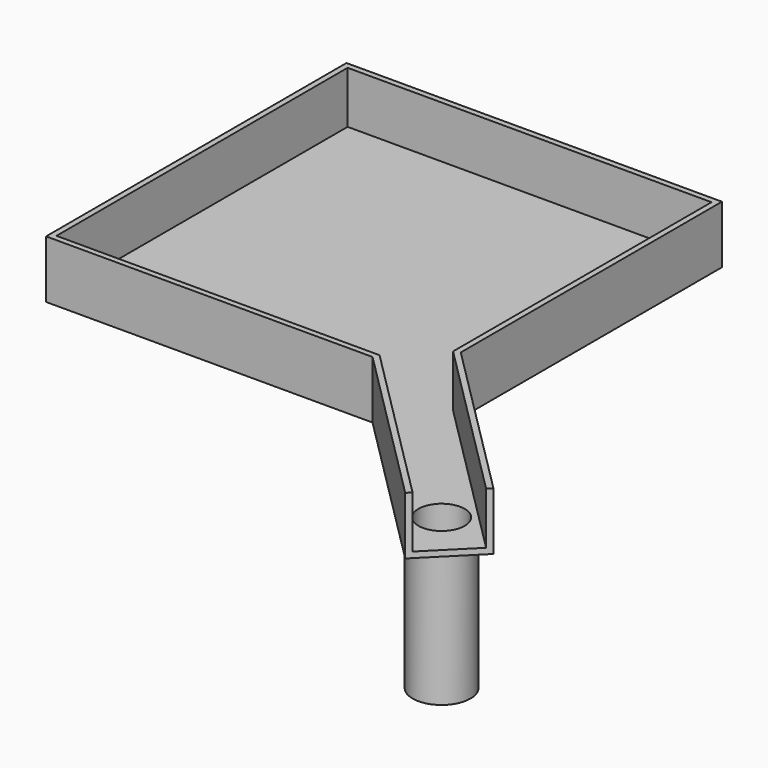
from build123d import *

# Parameters (mm, degrees)
F0_W           = 65
F0_H           = 65
F1_DEPTH       = 10
F2_T           = -1
F6_DEPTH       = 10.0380592229
F6_DEPTH_BACK  = 30
F8_DEPTH       = 64.9
F8_DEPTH_BACK  = 36.001
F9_R           = 5
F10_DEPTH      = 25
F10_DEPTH_BACK = 1
F11_R          = 4
F12_DEPTH      = 1
F12_DEPTH_BACK = 22.5


with BuildPart() as f1:
    # F0 (on Top) → F1 (new body)
    with BuildSketch(Plane.XY):
        Rectangle(F0_W, F0_H)
    extrude(amount=F1_DEPTH)

    # F2
    f2_openings = [f1.faces().sort_by_distance(p)[0] for p in [
        (0, 0, 10),
    ]]
    offset(amount=F2_T, openings=f2_openings)

    # F5 (on face) → F6 (join, two sides)
    with BuildSketch(Plane(origin=(35.3553390593, -35.3553390593, 0), x_dir=(0.7071067812, 0.7071067812, 0), z_dir=(0.7071067812, -0.7071067812, 0))) as f6_sk:
        Polygon((6, 10), (5, 10), (5, 1), (-5, 1), (-5, 10), (-6, 10), (-6, 0), (6, 0), align=None)
    extrude(amount=-F6_DEPTH)
    extrude(f6_sk.sketch, amount=F6_DEPTH_BACK)

    # F7 (on face) → F8 (cut, two sides)
    with BuildSketch(Plane(origin=(35.3553390593, -35.3553390593, 0), x_dir=(0.7071067812, 0.7071067812, 0), z_dir=(0.7071067812, -0.7071067812, 0))) as f8_sk:
        Polygon((0, 10), (-5, 10), (-5, 1), (5, 1), (5, 10), align=None)
    extrude(amount=-F8_DEPTH, mode=Mode.SUBTRACT)
    extrude(f8_sk.sketch, amount=F8_DEPTH_BACK, mode=Mode.SUBTRACT)

    # F9 (on Top) → F10 (join, two sides)
    with BuildSketch(Plane.XY) as f10_sk:
        with Locations((49.8375721066, -49.8375721066)):
            Circle(F9_R)
    extrude(amount=-F10_DEPTH)
    extrude(f10_sk.sketch, amount=F10_DEPTH_BACK)

    # F11 (on Top) → F12 (cut, two sides)
    with BuildSketch(Plane.XY) as f12_sk:
        with Locations((49.8375721066, -49.8375721066)):
            Circle(F11_R)
    extrude(amount=F12_DEPTH, mode=Mode.SUBTRACT)
    extrude(f12_sk.sketch, amount=-F12_DEPTH_BACK, mode=Mode.SUBTRACT)


solid = f1.part
